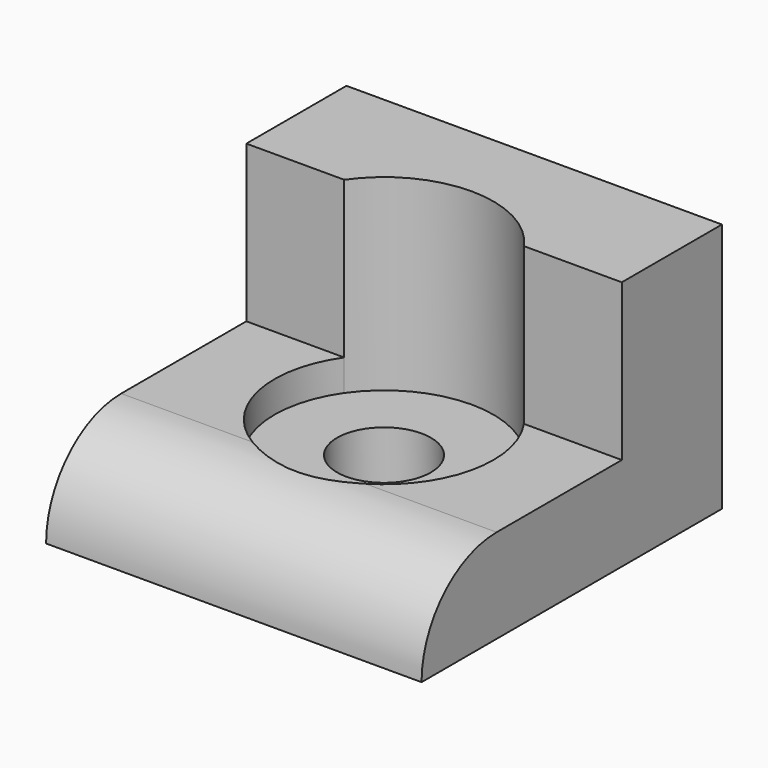
from build123d import *

# Parameters (mm, degrees)
F0_W     = 12
F0_H     = 12
F0_R     = 1.5
F1_DEPTH = 3
F2_W     = 12
F2_H     = 4
F3_DEPTH = 5
F5_R     = 2.99999
F6_DEPTH = 6


# Not quite as in the source:
# - a fillet or chamfer is up to 0.001 mm smaller than in the source, because OpenCascade refuses the exact size


with BuildPart() as f1:
    # F0 (on Top) → F1 (new body)
    with BuildSketch(Plane.XY):
        Rectangle(F0_W, F0_H)
        Circle(F0_R, mode=Mode.SUBTRACT)
    extrude(amount=F1_DEPTH)

    # F2 (on face) → F3 (join)
    with BuildSketch(Plane.XY.offset(3)):
        with Locations((0, 4)):
            Rectangle(F2_W, F2_H)
    extrude(amount=F3_DEPTH)

    # F5 (radius 3 in the source; OpenCascade refuses exactly that, so slightly less here)
    f5_edges = [f1.edges().sort_by_distance(p)[0] for p in [
        (0, -6, 3),
    ]]
    fillet(f5_edges, radius=F5_R)

    # F4 (on face) → F6 (cut)
    with BuildSketch(Plane.XY.offset(8)):
        with BuildLine():
            ThreePointArc((-2.8722813233, 2), (-1.0480971731, -3.3393850206), (3.5, 0))
            ThreePointArc((3.5, 0), (3.3393850206, 1.0480971731), (2.8722813233, 2))
            Line((2.8722813233, 2), (-2.8722813233, 2))
        make_face()
        with BuildLine():
            Line((-2.8722813233, 2), (2.8722813233, 2))
            ThreePointArc((2.8722813233, 2), (0, 3.5), (-2.8722813233, 2))
        make_face()
    extrude(amount=-F6_DEPTH, mode=Mode.SUBTRACT)


solid = f1.part
